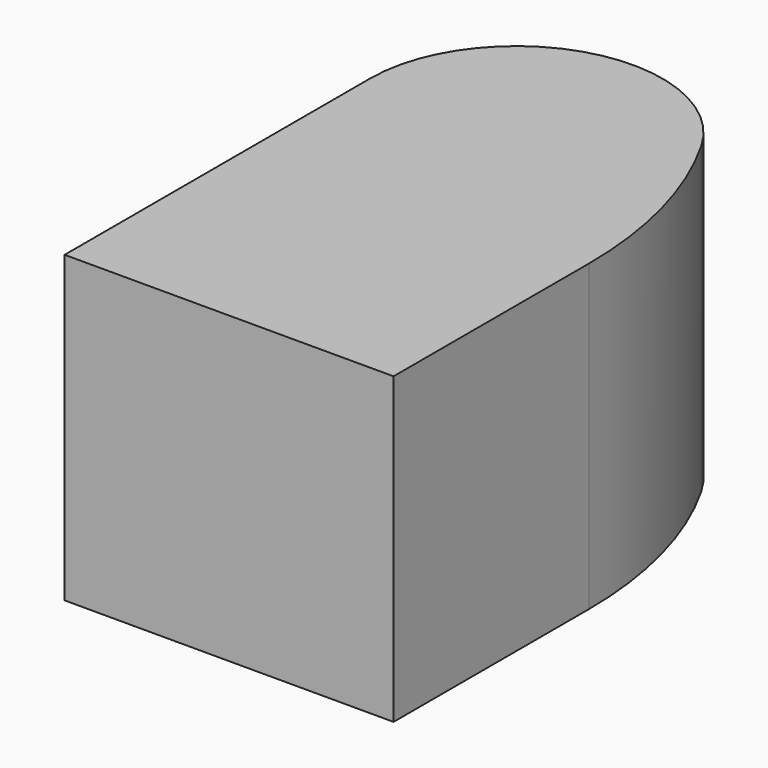
from build123d import *

# Parameters (mm, degrees)
F0_W        = 50.8
F0_H        = 101.6
F1_DEPTH    = 46.99
F2_T1_DEPTH = 366.5870593472
F3_R        = 22.587582604


# Not quite as in the source:
# - a fillet or chamfer that OpenCascade refuses, or shapes differently, is made with other operations: its cross-section is extruded or revolved along the edge and cut away or added


with BuildPart() as f1:
    # F0 (on Top) → F1 (new body)
    with BuildSketch(Plane.XY):
        with Locations((87.8112020218, -9.4523200796)):
            Rectangle(F0_W, F0_H)
    extrude(amount=F1_DEPTH)

    # F2: fillet of radius 65.6134961982 on 1 edges, made by hand

    # F2_s2 → F2_t1 (cut)
    with BuildSketch(Plane.XY.offset(-159.7985296736)):
        with BuildLine():
            ThreePointArc((62.4112020218, 41.3476799204), (98.964505217, 18.2520699738), (113.2112020218, -22.571731949))
            Line((113.2112020218, -22.571731949), (113.2112020218, 41.3476799204))
            Line((113.2112020218, 41.3476799204), (62.4112020218, 41.3476799204))
        make_face()
    extrude(amount=F2_T1_DEPTH, mode=Mode.SUBTRACT)

    # F3
    f3_edges = [f1.edges().sort_by_distance(p)[0] for p in [
        (62.411202, 41.34768, 23.495),
    ]]
    fillet(f3_edges, radius=F3_R)


solid = f1.part
